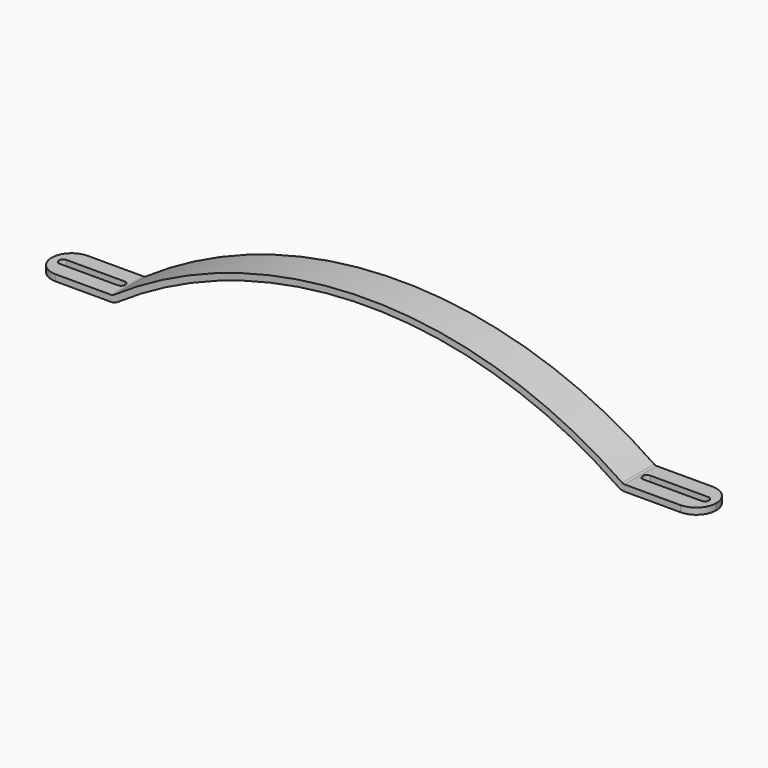
from build123d import *

# Parameters (mm, degrees)
F1_DEPTH = 19
F3_DEPTH = 25
F6_DEPTH = 6.001


# Not quite as in the source:
# - a pattern or mirror of a feature is missing from the dataset's text; its kind, count and spacing are read off the source's solid


with BuildPart() as f1:
    # F0 (on Front) → F1 (new body, symmetric)
    with BuildSketch(Plane.XZ):
        with BuildLine():
            ThreePointArc((-237.8384793929, 1.7578850393), (0, 75.589056691), (237.8384793929, 1.7578850393))
            ThreePointArc((237.8384793929, 1.7578850393), (240.5366038546, 0.4495772448), (243.5013003309, 0))
            Line((243.5013003309, 0), (315.377, 0))
            Line((315.377, 0), (315.377, 6))
            Line((315.377, 6), (243.5013003309, 6))
            ThreePointArc((243.5013003309, 6), (242.3154217403, 6.1798308979), (241.2361719557, 6.7031540157))
            ThreePointArc((241.2361719557, 6.7031540157), (0, 81.589056691), (-241.2361719557, 6.7031540157))
            ThreePointArc((-241.2361719557, 6.7031540157), (-242.3154217403, 6.1798308979), (-243.5013003309, 6))
            Line((-243.5013003309, 6), (-315.377, 6))
            Line((-315.377, 6), (-315.377, 0))
            Line((-315.377, 0), (-243.5013003309, 0))
            ThreePointArc((-243.5013003309, 0), (-240.5366038546, 0.4495772448), (-237.8384793929, 1.7578850393))
        make_face()
    extrude(amount=F1_DEPTH, both=True)

    # F2 (on face) → F3 (cut)
    with BuildSketch(Plane(origin=(0, 0, 0), x_dir=(1, 0, 0), z_dir=(0, 0, -1))):
        with BuildLine():
            Line((315.3777926865, -19), (315.3777926865, 0))
            ThreePointArc((315.3777926865, 0), (309.812821529, -13.4350288425), (296.3777926865, -19))
            Line((296.3777926865, -19), (315.3777926865, -19))
        make_face()
        with BuildLine():
            Line((315.3777926865, 19), (296.3777926865, 19))
            ThreePointArc((296.3777926865, 19), (309.812821529, 13.4350288425), (315.3777926865, 0))
            Line((315.3777926865, 0), (315.3777926865, 19))
        make_face()
    f3 = extrude(amount=-F3_DEPTH, mode=Mode.SUBTRACT)

    # F3_copies: F3 across plane
    add(f3.mirror(Plane(origin=(0, 0, 0), x_dir=(0, 0, -1), z_dir=(-1, 0, 0))), mode=Mode.SUBTRACT)

    # F5 (on offset) → F6 (cut, through all)
    with BuildSketch(Plane.XY.offset(6)):
        with BuildLine():
            ThreePointArc((304.4798749685, -4), (308.4798749685, 0), (304.4798749685, 4))
            Line((304.4798749685, 4), (249.4798749685, 4))
            ThreePointArc((249.4798749685, 4), (245.4798749685, 0), (249.4798749685, -4))
            Line((249.4798749685, -4), (304.4798749685, -4))
        make_face()
    f6 = extrude(amount=-F6_DEPTH, mode=Mode.SUBTRACT)

    # F6_copies: F6 across plane
    add(f6.mirror(Plane(origin=(0, 0, 0), x_dir=(0, 0, -1), z_dir=(-1, 0, 0))), mode=Mode.SUBTRACT)


solid = f1.part
